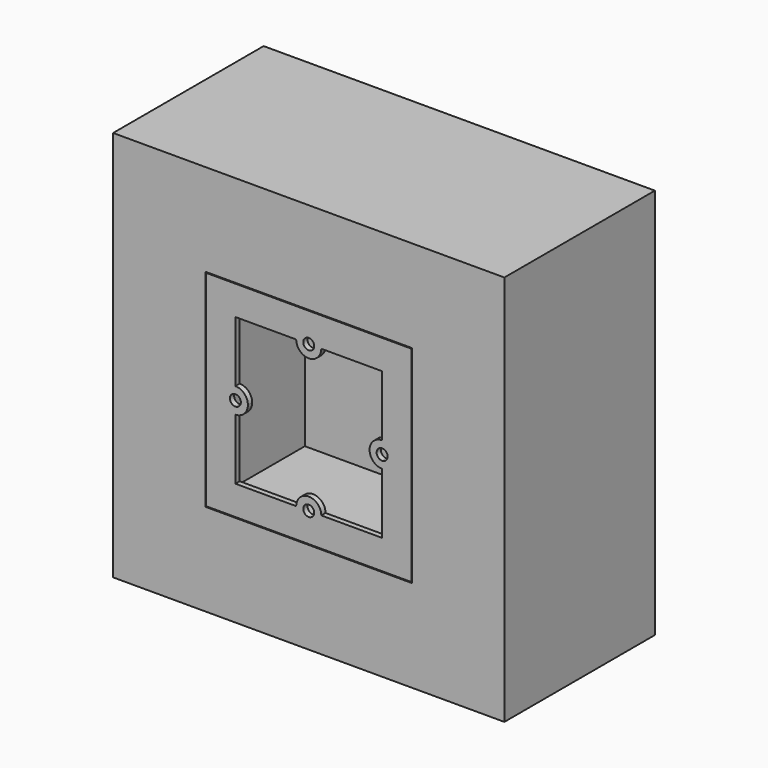
from build123d import *

# Parameters (mm, degrees)
F1_W     = 83.185
F1_H     = 83.185
F1_W_2   = 70.612
F1_H_2   = 70.612
F2_DEPTH = 2.159
F0_W     = 158.4607362747
F0_H     = 158.4607362747
F0_W_2   = 83.82
F0_H_2   = 83.82
F0_W_3   = 70.612
F0_H_3   = 70.612
F3_DEPTH = 76.2
F4_DEPTH = 2.159
F5_DEPTH = 42.164


with BuildPart() as f2:
    # F1 (on face) → F2 (new body)
    with BuildSketch(Plane.XZ):
        Rectangle(F1_W, F1_H)
        Rectangle(F1_W_2, F1_H_2, mode=Mode.SUBTRACT)
        Rectangle(F1_W_2, F1_H_2)
        with BuildLine():
            Line((5.08, 29.718), (29.718, 29.718))
            Line((29.718, 29.718), (29.718, 5.08))
            ThreePointArc((29.718, 5.08), (33.3101024484, 3.5921024484), (34.798, 0))
            ThreePointArc((34.798, 0), (33.3101024484, -3.5921024484), (29.718, -5.08))
            Line((29.718, -5.08), (29.718, -29.718))
            Line((29.718, -29.718), (5.08, -29.718))
            ThreePointArc((5.08, -29.718), (0, -34.798), (-5.08, -29.718))
            Line((-5.08, -29.718), (-29.718, -29.718))
            Line((-29.718, -29.718), (-29.718, -5.08))
            ThreePointArc((-29.718, -5.08), (-34.798, 0), (-29.718, 5.08))
            Line((-29.718, 5.08), (-29.718, 29.718))
            Line((-29.718, 29.718), (-5.08, 29.718))
            ThreePointArc((-5.08, 29.718), (0, 34.798), (5.08, 29.718))
        make_face(mode=Mode.SUBTRACT)
        with BuildLine():
            Line((-29.718, 2.2225), (-29.718, 5.08))
            ThreePointArc((-29.718, 5.08), (-34.798, 0), (-29.718, -5.08))
            Line((-29.718, -5.08), (-29.718, -2.2225))
            ThreePointArc((-29.718, -2.2225), (-31.9405, 0), (-29.718, 2.2225))
        make_face()
        with BuildLine():
            ThreePointArc((-24.638, 0), (-26.1258975516, 3.5921024484), (-29.718, 5.08))
            Line((-29.718, 5.08), (-29.718, 2.2225))
            ThreePointArc((-29.718, 2.2225), (-28.1464551788, 1.5715448212), (-27.4955, 0))
            ThreePointArc((-27.4955, 0), (-28.1464551788, -1.5715448212), (-29.718, -2.2225))
            Line((-29.718, -2.2225), (-29.718, -5.08))
            ThreePointArc((-29.718, -5.08), (-26.1258975516, -3.5921024484), (-24.638, 0))
        make_face()
        with BuildLine():
            ThreePointArc((-5.08, 29.718), (0, 24.638), (5.08, 29.718))
            Line((5.08, 29.718), (2.2225, 29.718))
            ThreePointArc((2.2225, 29.718), (0, 27.4955), (-2.2225, 29.718))
            Line((-2.2225, 29.718), (-5.08, 29.718))
        make_face()
        with BuildLine():
            Line((2.2225, 29.718), (5.08, 29.718))
            ThreePointArc((5.08, 29.718), (0, 34.798), (-5.08, 29.718))
            Line((-5.08, 29.718), (-2.2225, 29.718))
            ThreePointArc((-2.2225, 29.718), (0, 31.9405), (2.2225, 29.718))
        make_face()
        with BuildLine():
            Line((29.718, 2.2225), (29.718, 5.08))
            ThreePointArc((29.718, 5.08), (24.638, 0), (29.718, -5.08))
            Line((29.718, -5.08), (29.718, -2.2225))
            ThreePointArc((29.718, -2.2225), (27.4955, 0), (29.718, 2.2225))
        make_face()
        with BuildLine():
            ThreePointArc((34.798, 0), (33.3101024484, 3.5921024484), (29.718, 5.08))
            Line((29.718, 5.08), (29.718, 2.2225))
            ThreePointArc((29.718, 2.2225), (31.2895448212, 1.5715448212), (31.9405, 0))
            ThreePointArc((31.9405, 0), (31.2895448212, -1.5715448212), (29.718, -2.2225))
            Line((29.718, -2.2225), (29.718, -5.08))
            ThreePointArc((29.718, -5.08), (33.3101024484, -3.5921024484), (34.798, 0))
        make_face()
        with BuildLine():
            ThreePointArc((-5.08, -29.718), (0, -34.798), (5.08, -29.718))
            Line((5.08, -29.718), (2.2225, -29.718))
            ThreePointArc((2.2225, -29.718), (0, -31.9405), (-2.2225, -29.718))
            Line((-2.2225, -29.718), (-5.08, -29.718))
        make_face()
        with BuildLine():
            Line((2.2225, -29.718), (5.08, -29.718))
            ThreePointArc((5.08, -29.718), (0, -24.638), (-5.08, -29.718))
            Line((-5.08, -29.718), (-2.2225, -29.718))
            ThreePointArc((-2.2225, -29.718), (0, -27.4955), (2.2225, -29.718))
        make_face()
    extrude(amount=-F2_DEPTH)


with BuildPart() as f3:
    # F0 (on Front) → F3 (new body)
    with BuildSketch(Plane.XZ):
        Rectangle(F0_W, F0_H)
        Rectangle(F0_W_2, F0_H_2, mode=Mode.SUBTRACT)
        Rectangle(F0_W_2, F0_H_2)
        Rectangle(F0_W_3, F0_H_3, mode=Mode.SUBTRACT)
        Rectangle(F0_W_3, F0_H_3)
    extrude(amount=-F3_DEPTH)

    # F0 (on Front) → F4 (cut)
    with BuildSketch(Plane.XZ):
        Rectangle(F0_W_2, F0_H_2)
        Rectangle(F0_W_3, F0_H_3, mode=Mode.SUBTRACT)
        Rectangle(F0_W_3, F0_H_3)
    extrude(amount=-F4_DEPTH, mode=Mode.SUBTRACT)

    # F0 (on Front) → F5 (cut)
    with BuildSketch(Plane.XZ):
        Rectangle(F0_W_3, F0_H_3)
    extrude(amount=-F5_DEPTH, mode=Mode.SUBTRACT)


solid = Compound([f2.part, f3.part])
